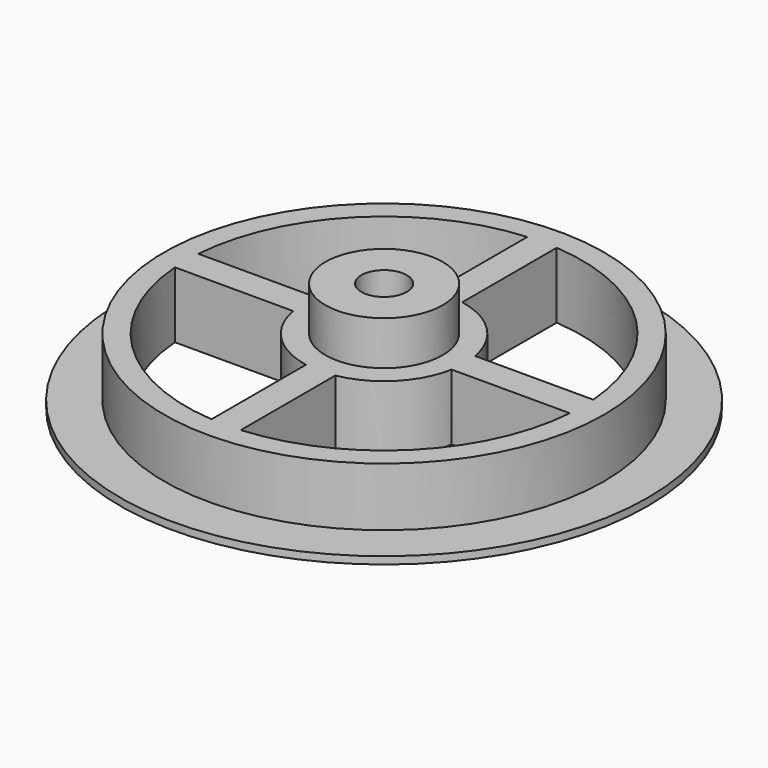
from build123d import *

# Parameters (mm, degrees)
F0_R     = 15
F1_DEPTH = 4
F2_R     = 18
F2_R_2   = 15
F3_DEPTH = 0.5
F4_R     = 4
F5_DEPTH = 3
F6_R     = 1.55
F7_DEPTH = 7.5
F9_DEPTH = 4.5


with BuildPart() as f1:
    # F0 (on Top) → F1 (new body)
    with BuildSketch(Plane.XY):
        Circle(F0_R)
    extrude(amount=F1_DEPTH)

    # F2 (on face) → F3 (join)
    with BuildSketch(Plane(origin=(0, 0, 0), x_dir=(1, 0, 0), z_dir=(0, 0, -1))):
        Circle(F2_R)
        Circle(F2_R_2, mode=Mode.SUBTRACT)
        Circle(F2_R_2)
    extrude(amount=F3_DEPTH)

    # F4 (on face) → F5 (join)
    with BuildSketch(Plane.XY.offset(4)):
        Circle(F4_R)
    extrude(amount=F5_DEPTH)

    # F6 (on face) → F7 (cut, through all)
    with BuildSketch(Plane.XY.offset(7)):
        Circle(F6_R)
    extrude(amount=-F7_DEPTH, mode=Mode.SUBTRACT)

    # F8 (on face) → F9 (cut, through all)
    with BuildSketch(Plane.XY.offset(4)):
        with BuildLine():
            ThreePointArc((-5.4083269132, 1), (-3.8890872965, 3.8890872965), (-1, 5.4083269132))
            Line((-1, 5.4083269132), (-1, 13.4629120178))
            ThreePointArc((-1, 13.4629120178), (-9.545941546, 9.545941546), (-13.4629120178, 1))
            Line((-13.4629120178, 1), (-5.4083269132, 1))
        make_face()
        with BuildLine():
            Line((1, 13.4629120178), (1, 5.4083269132))
            ThreePointArc((1, 5.4083269132), (3.8890872965, 3.8890872965), (5.4083269132, 1))
            Line((5.4083269132, 1), (13.4629120178, 1))
            ThreePointArc((13.4629120178, 1), (9.545941546, 9.545941546), (1, 13.4629120178))
        make_face()
        with BuildLine():
            Line((13.4629120178, -1), (5.4083269132, -1))
            ThreePointArc((5.4083269132, -1), (3.8890872965, -3.8890872965), (1, -5.4083269132))
            Line((1, -5.4083269132), (1, -13.4629120178))
            ThreePointArc((1, -13.4629120178), (9.545941546, -9.545941546), (13.4629120178, -1))
        make_face()
        with BuildLine():
            ThreePointArc((-1, -5.4083269132), (-3.8890872965, -3.8890872965), (-5.4083269132, -1))
            Line((-5.4083269132, -1), (-13.4629120178, -1))
            ThreePointArc((-13.4629120178, -1), (-9.545941546, -9.545941546), (-1, -13.4629120178))
            Line((-1, -13.4629120178), (-1, -5.4083269132))
        make_face()
    extrude(amount=-F9_DEPTH, mode=Mode.SUBTRACT)


solid = f1.part
